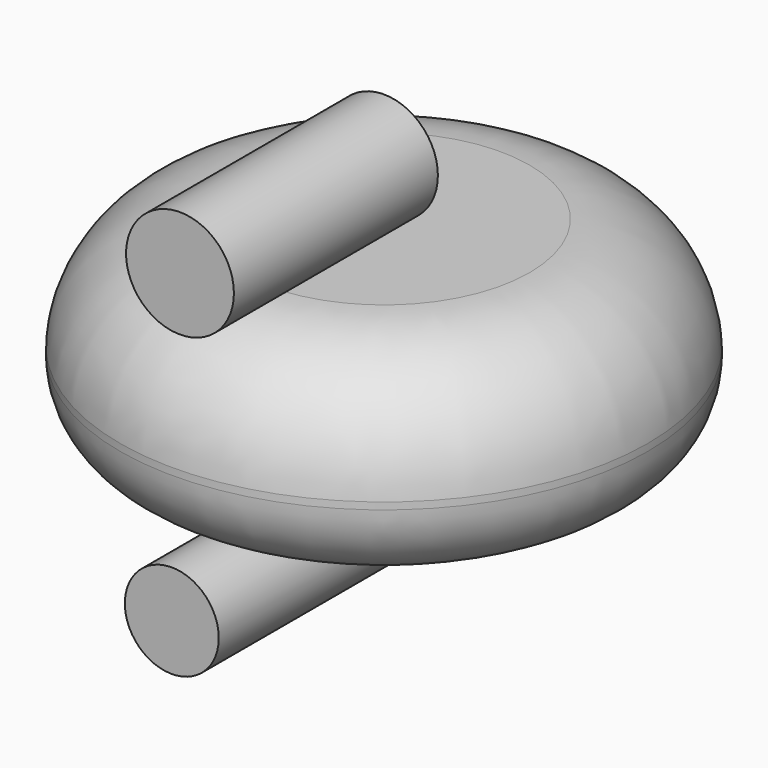
from build123d import *

# Parameters (mm, degrees)
F0_R     = 59.9383278597
F2_DEPTH = 25.4
F1_R     = 59.9383278597
F4_DEPTH = 19.7198782116
F5_R     = 18.1296998075
F6_R     = 12.2432091335
F7_DEPTH = 57.9018350691
F8_R     = 10.663859886
F9_DEPTH = 60.2239668369


# Not quite as in the source:
# - a fillet or chamfer that OpenCascade refuses, or shapes differently, is made with other operations: its cross-section is extruded or revolved along the edge and cut away or added


with BuildPart() as f2:
    # F0 (on Top) → F2 (new body)
    with BuildSketch(Plane.XY):
        Circle(F0_R)
    extrude(amount=F2_DEPTH)

    # F3: fillet of radius 26.9030647894 on 1 edges, made by hand

    # F3_s1 → F3_t2 (revolve, cut)
    with BuildSketch(Plane.XZ):
        with BuildLine():
            ThreePointArc((59.9383278597, 0), (51.5615722779, 18.044466314), (33.0772837381, 25.4))
            Line((33.0772837381, 25.4), (59.9383278597, 25.4))
            Line((59.9383278597, 25.4), (59.9383278597, 0))
        make_face()
    revolve(axis=Axis((0, 0, 25.4), (0, 0, 1)), mode=Mode.SUBTRACT)

    # F1 (on face) → F4 (join)
    with BuildSketch(Plane.XY):
        Circle(F1_R)
    extrude(amount=-F4_DEPTH)

    # F5
    f5_edges = [f2.edges().sort_by_distance(p)[0] for p in [
        (-59.938328, 0, -19.719878),
    ]]
    fillet(f5_edges, radius=F5_R)


with BuildPart() as f7:
    # F6 (on Front) → F7 (new body)
    with BuildSketch(Plane.XZ):
        with Locations((0, 38.0485132337)):
            Circle(F6_R)
    extrude(amount=F7_DEPTH)


with BuildPart() as f9:
    # F8 (on Front) → F9 (new body)
    with BuildSketch(Plane.XZ):
        with Locations((0, -30.4498225451)):
            Circle(F8_R)
    extrude(amount=F9_DEPTH)


solid = Compound([f2.part, f7.part, f9.part])
